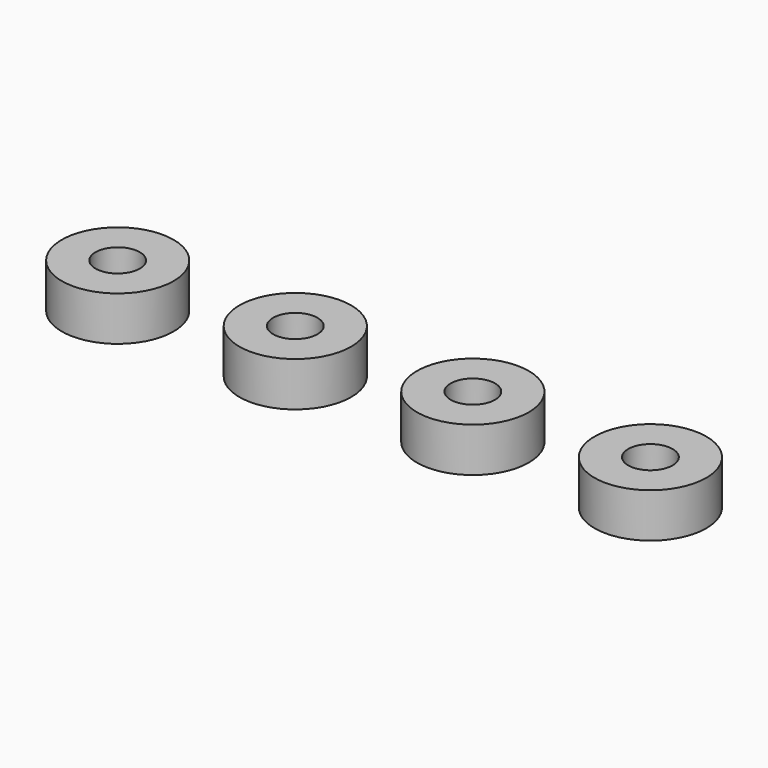
from build123d import *

# Parameters (mm, degrees)
F0_R     = 4
F0_R_2   = 1.5875
F1_DEPTH = 3.175


# Not quite as in the source:
# - a length typed as a fraction of an inch, garbled in the dataset ("3 / 203.2 mm" for 3/8 in), is restored


with BuildPart() as f1:
    # F0 (on Top) → F1 (new body)
    with BuildSketch(Plane.XY):
        Circle(F0_R)
        Circle(F0_R_2, mode=Mode.SUBTRACT)
    extrude(amount=F1_DEPTH)


with BuildPart() as f2_1:
    # F2: copy of F1
    add(f1.part.moved(Location((25.4, 0, 0))))


with BuildPart() as f3_1:
    # F3: copy of F2_1
    add(f2_1.part.moved(Location((-12.7, 0, 0))))


with BuildPart() as f4_1:
    # F4: copy of F1
    add(f1.part.moved(Location((-12.7, 0, 0))))


solid = Compound([f1.part, f2_1.part, f3_1.part, f4_1.part])
